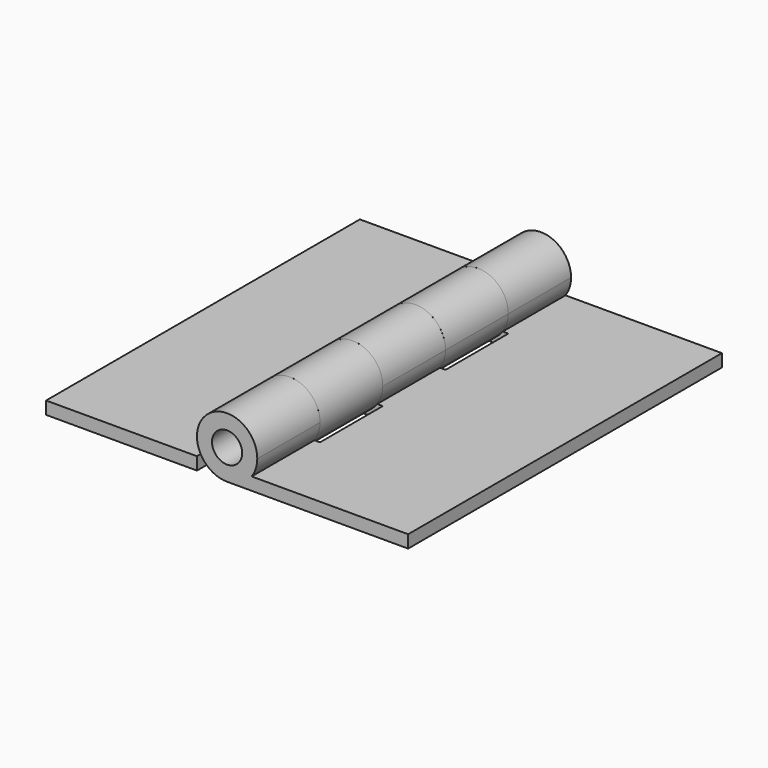
from build123d import *

# Parameters (mm, degrees)
F0_W      = 31.75
F0_H      = 82.55
F1_DEPTH  = 2.667
F2_W      = 16.51
F2_H      = 2.667
F3_DEPTH  = 6.35
F4_R      = 3.175
F5_DEPTH  = 16.51
F6_R      = 3.175
F7_DEPTH  = 16.51
F8_R      = 3.175
F9_DEPTH  = 16.51
F11_DEPTH = 2.667
F12_W     = 16.51
F12_H     = 2.667
F13_DEPTH = 6.35
F14_R     = 3.175
F15_DEPTH = 16.51
F16_R     = 3.175
F17_DEPTH = 16.51


with BuildPart() as f1:
    # F0 (on Top) → F1 (new body)
    with BuildSketch(Plane.XY):
        with Locations((15.875, 0)):
            Rectangle(F0_W, F0_H)
    extrude(amount=F1_DEPTH)

    # F2 (on face) → F3 (join)
    with BuildSketch(Plane(origin=(0, 0, 0), x_dir=(0, -1, 0), z_dir=(-1, 0, 0))):
        with Locations((-33.02, 1.3335)):
            Rectangle(F2_W, F2_H)
        with Locations((0, 1.3335)):
            Rectangle(F2_W, F2_H)
        with Locations((33.02, 1.3335)):
            Rectangle(F2_W, F2_H)
    extrude(amount=F3_DEPTH)

    # F4 (on face) → F5 (join, through all)
    with BuildSketch(Plane.XZ.offset(41.275)):
        with BuildLine():
            ThreePointArc((-1.177185389, 2.667), (-0.3014517122, 4.4167220557), (0, 6.35))
            ThreePointArc((0, 6.35), (-10.8401280605, 10.8401280605), (-6.35, 0))
            Line((-6.35, 0), (-6.35, 2.667))
            Line((-6.35, 2.667), (-1.177185389, 2.667))
        make_face()
        with Locations((-6.35, 6.35)):
            Circle(F4_R, mode=Mode.SUBTRACT)
    extrude(amount=-F5_DEPTH)

    # F6 (on face) → F7 (join, through all)
    with BuildSketch(Plane.XZ.offset(8.255)):
        with BuildLine():
            ThreePointArc((-1.177185389, 2.667), (-0.3014517122, 4.4167220557), (0, 6.35))
            ThreePointArc((0, 6.35), (-10.8401280605, 10.8401280605), (-6.35, 0))
            Line((-6.35, 0), (-6.35, 2.667))
            Line((-6.35, 2.667), (-1.177185389, 2.667))
        make_face()
        with Locations((-6.35, 6.35)):
            Circle(F6_R, mode=Mode.SUBTRACT)
    extrude(amount=-F7_DEPTH)

    # F8 (on face) → F9 (join, through all)
    with BuildSketch(Plane.XZ.offset(-24.765)):
        with BuildLine():
            ThreePointArc((-1.177185389, 2.667), (-0.3014517122, 4.4167220557), (0, 6.35))
            ThreePointArc((0, 6.35), (-10.8401280605, 10.8401280605), (-6.35, 0))
            Line((-6.35, 0), (-6.35, 2.667))
            Line((-6.35, 2.667), (-1.177185389, 2.667))
        make_face()
        with Locations((-6.35, 6.35)):
            Circle(F8_R, mode=Mode.SUBTRACT)
    extrude(amount=-F9_DEPTH)


with BuildPart() as f11:
    # F10 (on Top) → F11 (new body)
    with BuildSketch(Plane.XY):
        Polygon((-12.7, -40.005), (-12.7, 40.005), (-12.7, 41.275), (-44.45, 41.275), (-44.45, -41.275), (-12.7, -41.275), align=None)
    extrude(amount=F11_DEPTH)

    # F12 (on face) → F13 (join)
    with BuildSketch(Plane.YZ.offset(-12.7)):
        with Locations((-16.51, 1.3335)):
            Rectangle(F12_W, F12_H)
        with Locations((16.51, 1.3335)):
            Rectangle(F12_W, F12_H)
    extrude(amount=F13_DEPTH)

    # F14 (on face) → F15 (join, through all)
    with BuildSketch(Plane.XZ.offset(-24.765)):
        with BuildLine():
            ThreePointArc((-1.177185389, 2.667), (-0.3014517122, 4.4167220557), (0, 6.35))
            ThreePointArc((0, 6.35), (-10.8401280605, 10.8401280605), (-6.35, 0))
            ThreePointArc((-6.35, 0), (-3.4400644337, 0.705996545), (-1.177185389, 2.667))
        make_face()
        with Locations((-6.35, 6.35)):
            Circle(F14_R, mode=Mode.SUBTRACT)
    extrude(amount=F15_DEPTH)

    # F16 (on face) → F17 (join, through all)
    with BuildSketch(Plane(origin=(0, -24.765, 0), x_dir=(-1, 0, 0), z_dir=(0, 1, 0))):
        with BuildLine():
            ThreePointArc((6.35, 0), (10.8401280605, 1.8598719395), (12.7, 6.35))
            ThreePointArc((12.7, 6.35), (4.4167220557, 12.3985482878), (1.177185389, 2.667))
            ThreePointArc((1.177185389, 2.667), (3.4400644337, 0.705996545), (6.35, 0))
        make_face()
        with Locations((6.35, 6.35)):
            Circle(F16_R, mode=Mode.SUBTRACT)
    extrude(amount=F17_DEPTH)


solid = Compound([f1.part, f11.part])
